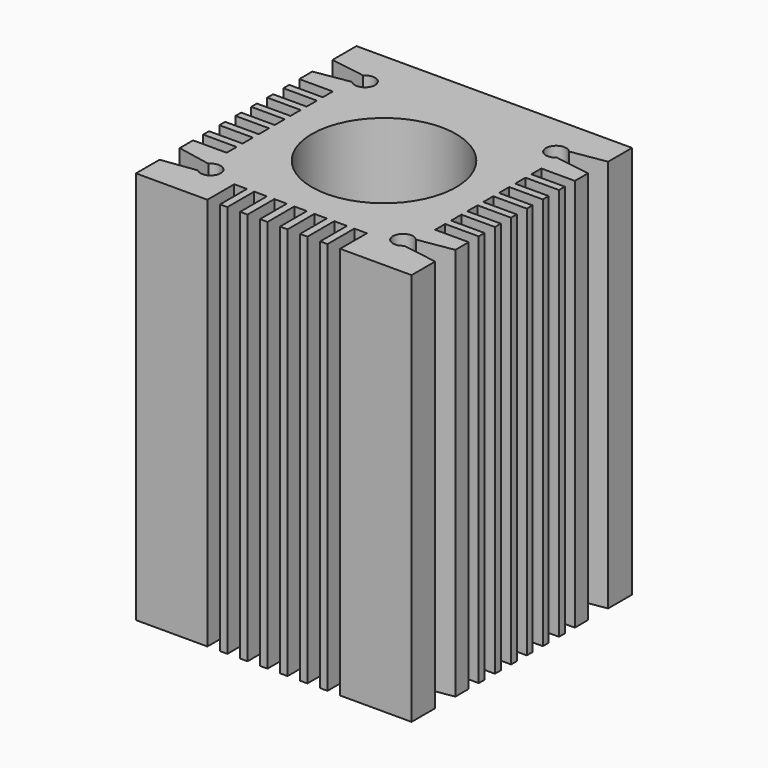
from build123d import *

# Parameters (mm, degrees)
F1_DEPTH = 49.53
F2_D     = 18.161
F4_D     = 3
F4_DEPTH = 7.366
F4_TIP   = 0.9012909285
F5_D     = 3
F5_DEPTH = 10.414
F5_TIP   = 0.9012909285
F6_D     = 5.334
F6_DEPTH = 7.874
F6_TIP   = 1.6024952709


# Not quite as in the source:
# - a feature of the source that left no trace in its solid (it failed there, or was rolled back) is left out


with BuildPart() as f1:
    # F0 (on Top) → F1 (new body)
    with BuildSketch(Plane.XY):
        with BuildLine():
            Line((-17.3533273419, -13.6358096689), (-17.3533273419, -17.3533273419))
            Line((-17.3533273419, -17.3533273419), (-8.3558009158, -17.3533273419))
            Line((-8.3558009158, -17.3533273419), (-8.3558009158, -13.1286343989))
            Line((-8.3558009158, -13.1286343989), (-6.7648564214, -13.1286343989))
            Line((-6.7648564214, -13.1286343989), (-6.7648564214, -17.3533273419))
            Line((-6.7648564214, -17.3533273419), (-5.8423760003, -17.3533273419))
            Line((-5.8423760003, -17.3533273419), (-5.8423760003, -13.1286343989))
            Line((-5.8423760003, -13.1286343989), (-4.2380622245, -13.1286343989))
            Line((-4.2380622245, -13.1286343989), (-4.2380622245, -17.3533273419))
            Line((-4.2380622245, -17.3533273419), (-3.3022125219, -17.3533273419))
            Line((-3.3022125219, -17.3533273419), (-3.3022125219, -13.1286343989))
            Line((-3.3022125219, -13.1286343989), (-1.7380065905, -13.1286343989))
            Line((-1.7380065905, -13.1286343989), (-1.7380065905, -17.3533273419))
            Line((-1.7380065905, -17.3533273419), (-0.7887876064, -17.3533273419))
            Line((-0.7887876064, -17.3533273419), (-0.7887876064, -13.1286343989))
            Line((-0.7887876064, -13.1286343989), (0.7887876064, -13.1286343989))
            Line((0.7887876064, -13.1286343989), (0.7887876064, -17.3533273419))
            Line((0.7887876064, -17.3533273419), (1.7380065905, -17.3533273419))
            Line((1.7380065905, -17.3533273419), (1.7380065905, -13.1286343989))
            Line((1.7380065905, -13.1286343989), (3.3022125219, -13.1286343989))
            Line((3.3022125219, -13.1286343989), (3.3022125219, -17.3533273419))
            Line((3.3022125219, -17.3533273419), (4.2380622245, -17.3533273419))
            Line((4.2380622245, -17.3533273419), (4.2380622245, -13.1286343989))
            Line((4.2380622245, -13.1286343989), (5.8423760003, -13.1286343989))
            Line((5.8423760003, -13.1286343989), (5.8423760003, -17.3533273419))
            Line((5.8423760003, -17.3533273419), (6.7648564214, -17.3533273419))
            Line((6.7648564214, -17.3533273419), (6.7648564214, -13.1286343989))
            Line((6.7648564214, -13.1286343989), (8.3558009158, -13.1286343989))
            Line((8.3558009158, -13.1286343989), (8.3558009158, -17.3533273419))
            Line((8.3558009158, -17.3533273419), (17.3533273419, -17.3533273419))
            Line((17.3533273419, -17.3533273419), (17.3533273419, -13.6358096689))
            Line((17.3533273419, -13.6358096689), (12.8737204648, -12.9246096689))
            ThreePointArc((12.8737204648, -12.9246096689), (10.7331515862, -11.9367520182), (12.9631890301, -11.1720096689))
            Line((12.9631890301, -11.1720096689), (17.3533273419, -10.4608096689))
            Line((17.3533273419, -10.4608096689), (17.3533273419, -8.3558009158))
            Line((17.3533273419, -8.3558009158), (13.1286343989, -8.3558009158))
            Line((13.1286343989, -8.3558009158), (13.1286343989, -6.7782257029))
            Line((13.1286343989, -6.7782257029), (17.3533273419, -6.7782257029))
            Line((17.3533273419, -6.7782257029), (17.3533273419, -5.8557452818))
            Line((17.3533273419, -5.8557452818), (13.1286343989, -5.8557452818))
            Line((13.1286343989, -5.8557452818), (13.1286343989, -4.224692943))
            Line((13.1286343989, -4.224692943), (17.3533273419, -4.224692943))
            Line((17.3533273419, -4.224692943), (17.3533273419, -3.3022125219))
            Line((17.3533273419, -3.3022125219), (13.1286343989, -3.3022125219))
            Line((13.1286343989, -3.3022125219), (13.1286343989, -1.6845294646))
            Line((13.1286343989, -1.6845294646), (17.3533273419, -1.6845294646))
            Line((17.3533273419, -1.6845294646), (17.3533273419, -0.7887876064))
            Line((17.3533273419, -0.7887876064), (13.1286343989, -0.7887876064))
            Line((13.1286343989, -0.7887876064), (13.1286343989, 0.7887876064))
            Line((13.1286343989, 0.7887876064), (17.3533273419, 0.7887876064))
            Line((17.3533273419, 0.7887876064), (17.3533273419, 1.6845294646))
            Line((17.3533273419, 1.6845294646), (13.1286343989, 1.6845294646))
            Line((13.1286343989, 1.6845294646), (13.1286343989, 3.3022125219))
            Line((13.1286343989, 3.3022125219), (17.3533273419, 3.3022125219))
            Line((17.3533273419, 3.3022125219), (17.3533273419, 4.224692943))
            Line((17.3533273419, 4.224692943), (13.1286343989, 4.224692943))
            Line((13.1286343989, 4.224692943), (13.1286343989, 5.8557452818))
            Line((13.1286343989, 5.8557452818), (17.3533273419, 5.8557452818))
            Line((17.3533273419, 5.8557452818), (17.3533273419, 6.7782257029))
            Line((17.3533273419, 6.7782257029), (13.1286343989, 6.7782257029))
            Line((13.1286343989, 6.7782257029), (13.1286343989, 8.3558009158))
            Line((13.1286343989, 8.3558009158), (17.3533273419, 8.3558009158))
            Line((17.3533273419, 8.3558009158), (17.3533273419, 10.414))
            Line((17.3533273419, 10.414), (12.8887263902, 11.1252))
            ThreePointArc((12.8887263902, 11.1252), (10.7559013561, 12.1292367927), (12.9912280955, 12.8778))
            Line((12.9912280955, 12.8778), (17.3533273419, 13.589))
            Line((17.3533273419, 13.589), (17.3533273419, 17.3533273419))
            Line((17.3533273419, 17.3533273419), (-17.3533273419, 17.3533273419))
            Line((-17.3533273419, 17.3533273419), (-17.3533273419, 13.589))
            Line((-17.3533273419, 13.589), (-12.9207378963, 12.8778))
            ThreePointArc((-12.9207378963, 12.8778), (-10.7315, 12.0015), (-12.9207378963, 11.1252))
            Line((-12.9207378963, 11.1252), (-17.3533273419, 10.414))
            Line((-17.3533273419, 10.414), (-17.3533273419, 8.3558009158))
            Line((-17.3533273419, 8.3558009158), (-13.1286343989, 8.3558009158))
            Line((-13.1286343989, 8.3558009158), (-13.1286343989, 6.7782257029))
            Line((-13.1286343989, 6.7782257029), (-17.3533273419, 6.7782257029))
            Line((-17.3533273419, 6.7782257029), (-17.3533273419, 5.8557452818))
            Line((-17.3533273419, 5.8557452818), (-13.1286343989, 5.8557452818))
            Line((-13.1286343989, 5.8557452818), (-13.1286343989, 4.224692943))
            Line((-13.1286343989, 4.224692943), (-17.3533273419, 4.224692943))
            Line((-17.3533273419, 4.224692943), (-17.3533273419, 3.3022125219))
            Line((-17.3533273419, 3.3022125219), (-13.1286343989, 3.3022125219))
            Line((-13.1286343989, 3.3022125219), (-13.1286343989, 1.6845294646))
            Line((-13.1286343989, 1.6845294646), (-17.3533273419, 1.6845294646))
            Line((-17.3533273419, 1.6845294646), (-17.3533273419, 0.7887876064))
            Line((-17.3533273419, 0.7887876064), (-13.1286343989, 0.7887876064))
            Line((-13.1286343989, 0.7887876064), (-13.1286343989, -0.7887876064))
            Line((-13.1286343989, -0.7887876064), (-17.3533273419, -0.7887876064))
            Line((-17.3533273419, -0.7887876064), (-17.3533273419, -1.6845294646))
            Line((-17.3533273419, -1.6845294646), (-13.1286343989, -1.6845294646))
            Line((-13.1286343989, -1.6845294646), (-13.1286343989, -3.3022125219))
            Line((-13.1286343989, -3.3022125219), (-17.3533273419, -3.3022125219))
            Line((-17.3533273419, -3.3022125219), (-17.3533273419, -4.224692943))
            Line((-17.3533273419, -4.224692943), (-13.1286343989, -4.224692943))
            Line((-13.1286343989, -4.224692943), (-13.1286343989, -5.8557452818))
            Line((-13.1286343989, -5.8557452818), (-17.3533273419, -5.8557452818))
            Line((-17.3533273419, -5.8557452818), (-17.3533273419, -6.7782257029))
            Line((-17.3533273419, -6.7782257029), (-13.1286343989, -6.7782257029))
            Line((-13.1286343989, -6.7782257029), (-13.1286343989, -8.3558009158))
            Line((-13.1286343989, -8.3558009158), (-17.3533273419, -8.3558009158))
            Line((-17.3533273419, -8.3558009158), (-17.3533273419, -10.4608096689))
            Line((-17.3533273419, -10.4608096689), (-13.0901890301, -11.2990096689))
            ThreePointArc((-13.0901890301, -11.2990096689), (-10.8601515862, -12.0637520182), (-13.0007204648, -13.0516096689))
            Line((-13.0007204648, -13.0516096689), (-17.3533273419, -13.6358096689))
        make_face()
    extrude(amount=F1_DEPTH)

    # F2 (through all)
    with Locations(Plane(origin=(0, 0, 0), x_dir=(1, 0, 0), z_dir=(0, 0, -1))):
        with Locations((0, 0)):
            Hole(F2_D / 2)

    # F4
    with Locations(Plane(origin=(0, 17.3533273419, 0), x_dir=(-1, 0, 0), z_dir=(0, 1, 0))):
        with Locations((0.033583874, 44.765), (0.033583874, 4.765)):
            Hole(F4_D / 2, depth=F4_DEPTH)
            with Locations((0, 0, -(F4_DEPTH + F4_TIP / 2))):  # 118° drill point
                Cone(0, F4_D / 2, F4_TIP, mode=Mode.SUBTRACT)

    # F5
    with Locations(Plane(origin=(0, 17.3533273419, 0), x_dir=(-1, 0, 0), z_dir=(0, 1, 0))):
        with Locations((8.033583874, 44.765), (8.033583874, 4.765), (-7.966416126, 4.765), (-7.966416126, 44.765)):
            Hole(F5_D / 2, depth=F5_DEPTH)
            with Locations((0, 0, -(F5_DEPTH + F5_TIP / 2))):  # 118° drill point
                Cone(0, F5_D / 2, F5_TIP, mode=Mode.SUBTRACT)

    # F6
    with Locations(Plane(origin=(0, 17.3533273419, 0), x_dir=(-1, 0, 0), z_dir=(0, 1, 0))):
        with Locations((0.033583874, 24.765)):
            Hole(F6_D / 2, depth=F6_DEPTH)
            with Locations((0, 0, -(F6_DEPTH + F6_TIP / 2))):  # 118° drill point
                Cone(0, F6_D / 2, F6_TIP, mode=Mode.SUBTRACT)


solid = f1.part
